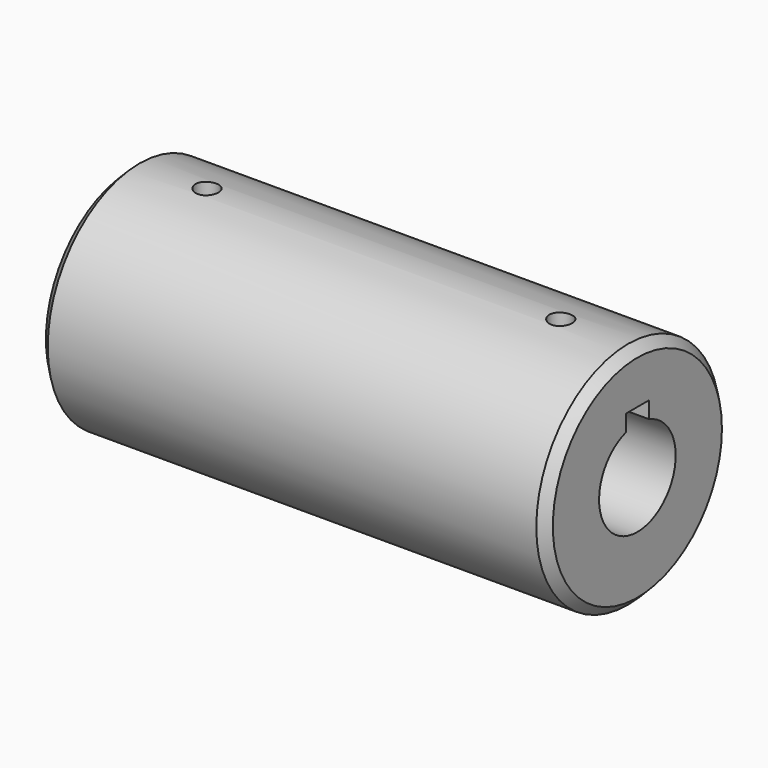
from build123d import *

# Parameters (mm, degrees)
F0_R     = 19.05
F1_DEPTH = 42.037
F4_D     = 3.7973
F4_DEPTH = 12
F4_START = 0.0948523
F4_TIP   = 1.1408240143
F5_SIZE  = 1.524


with BuildPart() as f1:
    # F0 (on Right) → F1 (new body, symmetric)
    with BuildSketch(Plane.YZ):
        Circle(F0_R)
        with BuildLine():
            ThreePointArc((2.38125, 7.5718924112), (0, -7.9375), (-2.38125, 7.5718924112))
            Line((-2.38125, 7.5718924112), (-2.38125, 10.31875))
            Line((-2.38125, 10.31875), (2.38125, 10.31875))
            Line((2.38125, 10.31875), (2.38125, 7.5718924112))
        make_face(mode=Mode.SUBTRACT)
    extrude(amount=F1_DEPTH, both=True)

    # F4
    # its depths count from where the whole tool has entered the part; down to there all is cleared
    with Locations(Plane.XY.offset(19.05).offset(-F4_START)):
        with Locations((29.337, 0), (-29.337, 0)):
            Hole(F4_D / 2, depth=F4_DEPTH)
            with Locations((0, 0, -(F4_DEPTH + F4_TIP / 2))):  # 118° drill point
                Cone(0, F4_D / 2, F4_TIP, mode=Mode.SUBTRACT)

    # F5
    f5_edges = [f1.edges().sort_by_distance(p)[0] for p in [
        (42.037, -19.05, 0),
        (-42.037, -19.05, 0),
    ]]
    chamfer(f5_edges, length=F5_SIZE)


solid = f1.part
